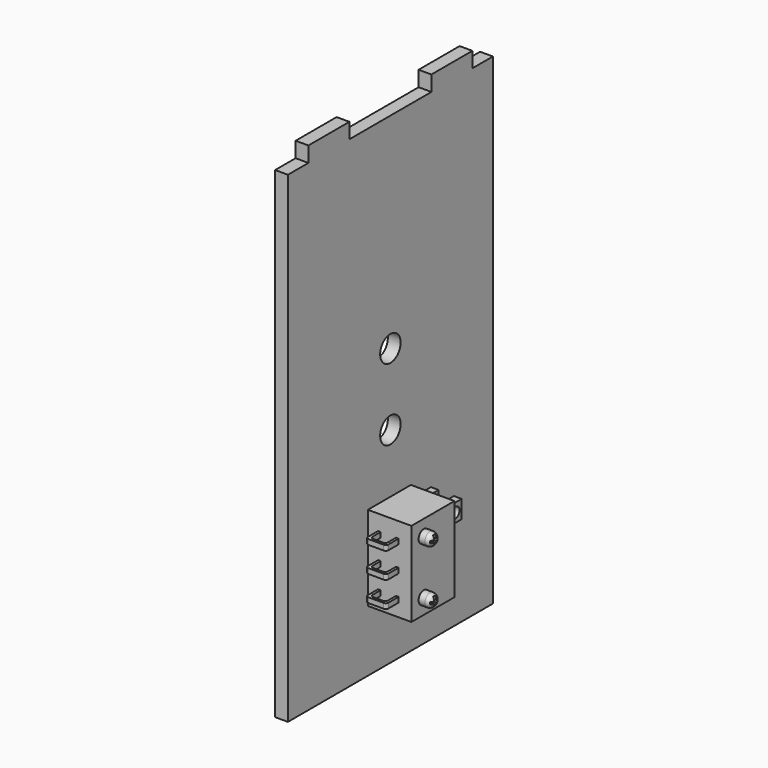
from build123d import *

# Parameters (mm, degrees)
F0_W      = 50
F0_H      = 94
F1_DEPTH  = 2.5
F2_W      = 2.5
F2_H      = 10
F3_DEPTH  = 3
F4_R      = 2.5
F5_DEPTH  = 25
F6_W      = 10.5
F6_H      = 16.5188284865
F7_DEPTH  = 8.5
F8_W      = 4
F8_H      = 1
F9_DEPTH  = 3
F11_DEPTH = 82.4821715135
F12_R     = 0.5
F13_R     = 1.25
F14_DEPTH = 2.25
F16_DEPTH = 2
F18_W     = 1.5
F18_H     = 3.5
F19_DEPTH = 3
F20_R     = 1
F21_DEPTH = 6


# Not quite as in the source:
# - a fillet or chamfer that OpenCascade refuses, or shapes differently, is made with other operations: its cross-section is extruded or revolved along the edge and cut away or added


with BuildPart() as f1:
    # F0 (on Right) → F1 (new body)
    with BuildSketch(Plane.YZ):
        with Locations((25, 47)):
            Rectangle(F0_W, F0_H)
    extrude(amount=F1_DEPTH)

    # F2 (on face) → F3 (join)
    with BuildSketch(Plane.XY.offset(94)):
        with Locations((1.25, 40)):
            Rectangle(F2_W, F2_H)
        with Locations((1.25, 10)):
            Rectangle(F2_W, F2_H)
    extrude(amount=F3_DEPTH)

    # F4 (on face) → F5 (cut)
    with BuildSketch(Plane.YZ.offset(2.5)):
        with Locations((25, 40)):
            Circle(F4_R)
        with Locations((25, 54)):
            Circle(F4_R)
    extrude(amount=-F5_DEPTH, mode=Mode.SUBTRACT)

    # F6 (on face) → F7 (join)
    with BuildSketch(Plane.YZ.offset(2.5)):
        with Locations((24.75, 20.2594142432)):
            Rectangle(F6_W, F6_H)
    extrude(amount=F7_DEPTH)

    # F8 (on face) → F9 (join)
    with BuildSketch(Plane.XZ.offset(-19.5)):
        with Locations((6.5, 25.0188284865)):
            Rectangle(F8_W, F8_H)
        with Locations((6.5, 20.0188284865)):
            Rectangle(F8_W, F8_H)
        with Locations((6.5, 15.0188284865)):
            Rectangle(F8_W, F8_H)
    extrude(amount=F9_DEPTH)

    # F10 (on face) → F11 (cut, through all)
    with BuildSketch(Plane(origin=(0, 0, 14.5188284865), x_dir=(1, 0, 0), z_dir=(0, 0, -1))):
        with BuildLine():
            Line((5, -17.5), (5, -19.5))
            Line((5, -19.5), (8, -19.5))
            Line((8, -19.5), (8, -17.5))
            ThreePointArc((8, -17.5), (7.8535533906, -17.1464466094), (7.5, -17))
            Line((7.5, -17), (5.5, -17))
            ThreePointArc((5.5, -17), (5.1464466094, -17.1464466094), (5, -17.5))
        make_face()
    extrude(amount=-F11_DEPTH, mode=Mode.SUBTRACT)

    # F12
    f12_edges = [f1.edges().sort_by_distance(p)[0] for p in [
        (8.5, 16.5, 15.018828),
        (8.5, 16.5, 20.018828),
        (8.5, 16.5, 25.018828),
        (4.5, 16.5, 25.018828),
        (4.5, 16.5, 20.018828),
        (4.5, 16.5, 15.018828),
    ]]
    fillet(f12_edges, radius=F12_R)

    # F13 (on face) → F14 (join)
    with BuildSketch(Plane.YZ.offset(11)):
        with Locations((22.5, 25.5188284865)):
            Circle(F13_R)
        with Locations((22.5, 15)):
            Circle(F13_R)
    extrude(amount=F14_DEPTH)

    # F15 (on face) → F16 (cut)
    with BuildSketch(Plane.YZ.offset(13.25)):
        Polygon((22.2532600164, 25.2959672362), (22.2532600164, 24.5808176696), (22.7513108402, 24.5808176696), (22.7513108402, 25.2959672362), (23.51754345, 25.2959672362), (23.51754345, 25.7301647216), (22.7513108402, 25.7301647216), (22.7513108402, 26.4325458556), (22.2532600164, 26.4325458556), (22.2532600164, 25.7301647216), (21.5636510402, 25.7301647216), (21.5636510402, 25.2959672362), align=None)
        Polygon((22.2596314482, 14.7567068819), (22.2596314482, 14.0415573154), (22.757682272, 14.0415573154), (22.757682272, 14.7567068819), (23.5239148817, 14.7567068819), (23.5239148817, 15.1909043674), (22.757682272, 15.1909043674), (22.757682272, 15.8932855014), (22.2596314482, 15.8932855014), (22.2596314482, 15.1909043674), (21.5700224719, 15.1909043674), (21.5700224719, 14.7567068819), align=None)
    extrude(amount=-F16_DEPTH, mode=Mode.SUBTRACT)

    # F17: fillet of radius 1 on 2 edges, made by hand

    # F17_s1 → F17_t2 (revolve, cut)
    with BuildSketch(Plane.XY.offset(25.5188284865)):
        with BuildLine():
            ThreePointArc((12.25, 23.75), (12.9571067812, 23.4571067812), (13.25, 22.75))
            Line((13.25, 22.75), (13.25, 23.75))
            Line((13.25, 23.75), (12.25, 23.75))
        make_face()
    revolve(axis=Axis((13.25, 22.5, 25.5188284865), (1, 0, 0)), mode=Mode.SUBTRACT)

    # F17_s3 → F17_t4 (revolve, cut)
    with BuildSketch(Plane.XY.offset(15)):
        with BuildLine():
            ThreePointArc((12.25, 23.75), (12.9571067812, 23.4571067812), (13.25, 22.75))
            Line((13.25, 22.75), (13.25, 23.75))
            Line((13.25, 23.75), (12.25, 23.75))
        make_face()
    revolve(axis=Axis((13.25, 22.5, 15), (1, 0, 0)), mode=Mode.SUBTRACT)

    # F18 (on face) → F19 (join)
    with BuildSketch(Plane(origin=(0, 30, 0), x_dir=(-1, 0, 0), z_dir=(0, 1, 0))):
        with Locations((-9.25, 25.5901701748)):
            Rectangle(F18_W, F18_H)
        with Locations((-4.75, 25.6615988507)):
            Rectangle(F18_W, F18_H)
    extrude(amount=F19_DEPTH)

    # F20 (on face) → F21 (cut)
    with BuildSketch(Plane.YZ.offset(10)):
        with Locations((31.5, 25.5901701748)):
            Circle(F20_R)
    extrude(amount=-F21_DEPTH, mode=Mode.SUBTRACT)


solid = f1.part
